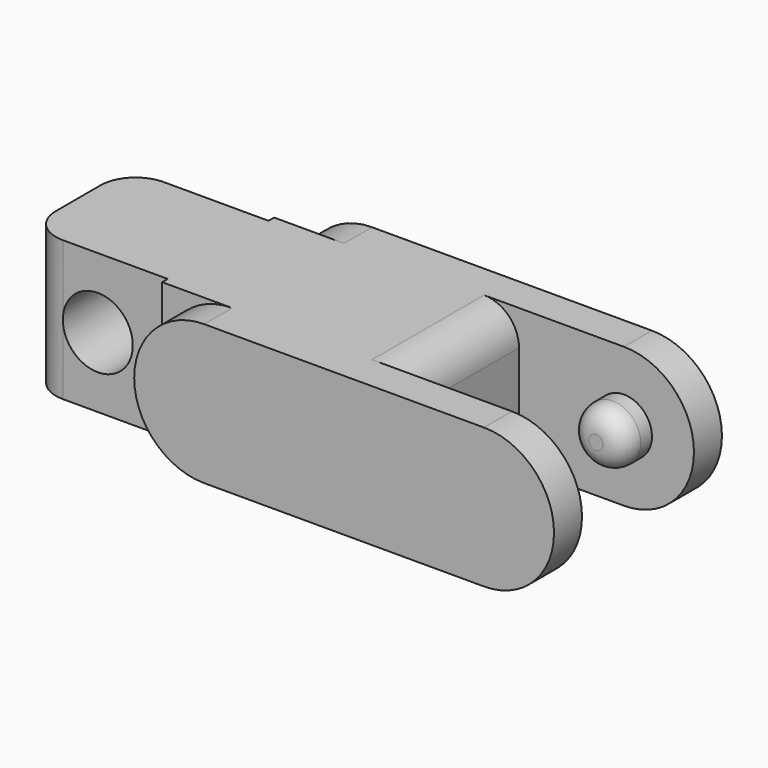
from build123d import *

# Parameters (mm, degrees)
F0_R      = 0.5
F1_DEPTH  = 2
F0_R_2    = 0.4
F2_DEPTH  = 0.5
F3_R      = 0.4
F4_DEPTH  = 0.5
F5_D      = 1
F6_DEPTH  = 0.5
F7_DEPTH  = 0.5
F8_R      = 0.3
F9_W      = 2
F9_H      = 0.1
F10_DEPTH = 25
F11_R     = 0.49999


# Not quite as in the source:
# - a fillet or chamfer is up to 0.001 mm smaller than in the source, because OpenCascade refuses the exact size
# - a feature names something its author has since deleted; it is built from what else it names


with BuildPart() as f1:
    # F0 (on Front) → F1 (new body)
    with BuildSketch(Plane.XZ):
        with BuildLine():
            Line((-1.5, -1.2454767711), (-1.5, -0.24940907))
            Line((-1.5, -0.24940907), (-4, -0.24940907))
            ThreePointArc((-4, -0.24940907), (-5, -1.24940907), (-4, -2.24940907))
            Line((-4, -2.24940907), (-1.5, -2.24940907))
            Line((-1.5, -2.24940907), (-1.5, -1.2454767711))
        make_face()
        with BuildLine():
            ThreePointArc((-4, -2.24940907), (-5, -1.24940907), (-4, -0.24940907))
            Line((-4, -0.24940907), (-7, -0.24940907))
            Line((-7, -0.24940907), (-7, -2.24940907))
            Line((-7, -2.24940907), (-4, -2.24940907))
        make_face()
        with Locations((-6, -1.24940907)):
            Circle(F0_R, mode=Mode.SUBTRACT)
        with Locations((-6, -1.24940907)):
            Circle(F0_R)
    extrude(amount=F1_DEPTH)

    # F0 (on Front) → F2 (join)
    with BuildSketch(Plane.XZ):
        with BuildLine():
            Line((-1.5, -1.2454767711), (-1.5, -0.24940907))
            Line((-1.5, -0.24940907), (-4, -0.24940907))
            ThreePointArc((-4, -0.24940907), (-5, -1.24940907), (-4, -2.24940907))
            Line((-4, -2.24940907), (-1.5, -2.24940907))
            Line((-1.5, -2.24940907), (-1.5, -1.2454767711))
        make_face()
        with BuildLine():
            Line((0, -0.24940907), (-1, -0.24940907))
            Line((-1, -0.24940907), (-1, -2.24940907))
            Line((-1, -2.24940907), (0, -2.24940907))
            ThreePointArc((0, -2.24940907), (1, -1.24940907), (0, -0.24940907))
        make_face()
        with Locations((0, -1.24940907)):
            Circle(F0_R_2, mode=Mode.SUBTRACT)
        Polygon((-1, -2.24940907), (-1, -0.24940907), (-1.5, -0.24940907), (-1.5, -1.2454767711), (-1.5, -2.24940907), align=None)
        with Locations((0, -1.24940907)):
            Circle(F0_R_2)
    extrude(amount=-F2_DEPTH)

    # F3 (on face) → F4 (join)
    with BuildSketch(Plane.XZ.offset(2)):
        with BuildLine():
            Line((-1.5, -2.24940907), (-1.5, -0.24940907))
            Line((-1.5, -0.24940907), (-4, -0.24940907))
            ThreePointArc((-4, -0.24940907), (-5, -1.24940907), (-4, -2.24940907))
            Line((-4, -2.24940907), (-1.5, -2.24940907))
        make_face()
        with BuildLine():
            Line((0, -0.24940907), (-1, -0.24940907))
            Line((-1, -0.24940907), (-1.5, -0.24940907))
            Line((-1.5, -0.24940907), (-1.5, -2.24940907))
            Line((-1.5, -2.24940907), (0, -2.24940907))
            ThreePointArc((0, -2.24940907), (1, -1.24940907), (0, -0.24940907))
        make_face()
        with Locations((0, -1.24940907)):
            Circle(F3_R, mode=Mode.SUBTRACT)
        with Locations((0, -1.24940907)):
            Circle(F3_R)
    extrude(amount=F4_DEPTH)

    # F5 (through all)
    with Locations(Plane(origin=(0, 0, 0), x_dir=(1, 0, 0), z_dir=(0, 1, 0))):
        with Locations((-6, 1.24940907)):
            Hole(F5_D / 2)

    # F0 (on Front) → F6 (join)
    with BuildSketch(Plane.XZ):
        with Locations((0, -1.24940907)):
            Circle(F0_R_2)
    extrude(amount=F6_DEPTH)

    # F3 (on face) → F7 (join)
    with BuildSketch(Plane.XZ.offset(2)):
        with Locations((0, -1.24940907)):
            Circle(F3_R)
    extrude(amount=-F7_DEPTH)

    # F8
    f8_edges = [f1.edges().sort_by_distance(p)[0] for p in [
        (-0.4, -0.5, -1.249409),
        (-0.4, -1.5, -1.249409),
    ]]
    fillet(f8_edges, radius=F8_R)

    # F9 (on face) → F10 (cut)
    with BuildSketch(Plane(origin=(0, 0, -2.24940907), x_dir=(1, 0, 0), z_dir=(0, 0, -1))):
        with Locations((-6, 1.95)):
            Rectangle(F9_W, F9_H)
        with Locations((-6, 0.05)):
            Rectangle(F9_W, F9_H)
    extrude(amount=-F10_DEPTH, mode=Mode.SUBTRACT)

    # F11 (radius 0.5 in the source; OpenCascade refuses exactly that, so slightly less here)
    f11_edges = [f1.edges().sort_by_distance(p)[0] for p in [
        (-7, -1.9, -1.249409),
        (-7, -0.1, -1.249409),
        (-1.5, -1, -0.249409),
        (-1.5, -1, -2.249409),
    ]]
    fillet(f11_edges, radius=F11_R)


solid = f1.part
